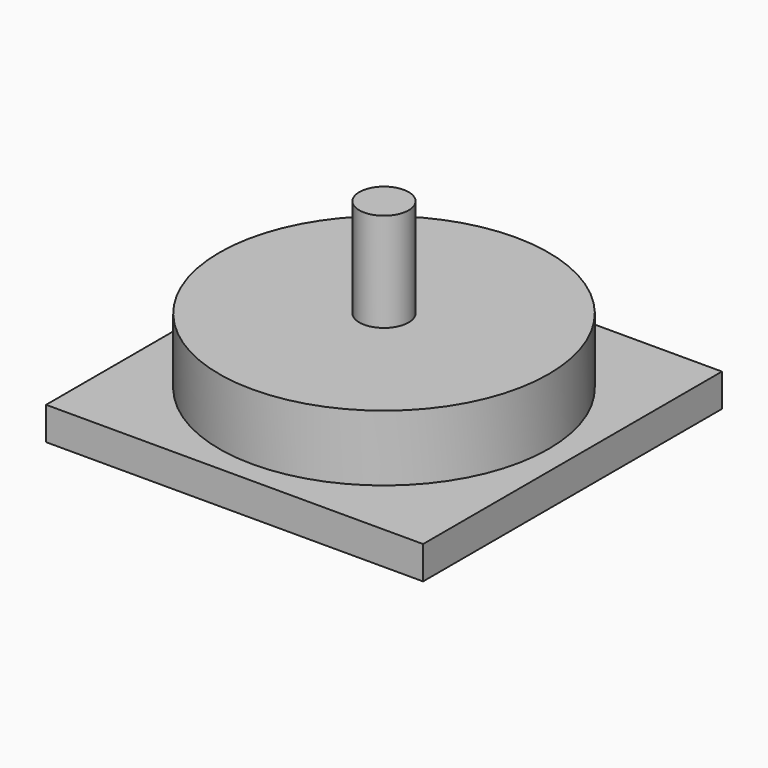
from build123d import *

# Parameters (mm, degrees)
F1_R         = 1.905
F2_DEPTH     = 12.7
F3_W         = 29.0826242417
F3_H         = 28.81863527
F4_DEPTH     = 2.54
F0_R         = 12.7
F5_DEPTH     = 5.08
F6_TEXT_SIZE = 25.5504752406
F7_DEPTH     = 2.54


# Not quite as in the source:
# - Text() gives the source's letters only with a copy of the font that has no kerning and outlines rounded to 1/6400 em; it was checked with that copy


with BuildPart() as f2:
    # F1 (on face) → F2 (new body)
    with BuildSketch(Plane.XY):
        Circle(F1_R)
    extrude(amount=F2_DEPTH)


with BuildPart() as f4:
    # F3 (on Top) → F4 (new body)
    with BuildSketch(Plane.XY):
        Rectangle(F3_W, F3_H)
    extrude(amount=-F4_DEPTH)

    # F6 (on face) → F7 (join)
    with BuildSketch(Plane(origin=(0, 0, -2.54), x_dir=(1, 0, 0), z_dir=(0, 0, -1))):
        with Locations((-12.2677572072, -8.6312917992)):
            Text('M', F6_TEXT_SIZE, font='Open Sans', font_style=FontStyle.BOLD, text_align=(TextAlign.LEFT, TextAlign.BOTTOM))
    extrude(amount=F7_DEPTH)


with BuildPart() as f5:
    # F0 (on Top) → F5 (new body)
    with BuildSketch(Plane.XY):
        Circle(F0_R)
    extrude(amount=F5_DEPTH)


solid = Compound([f2.part, f4.part, f5.part])
